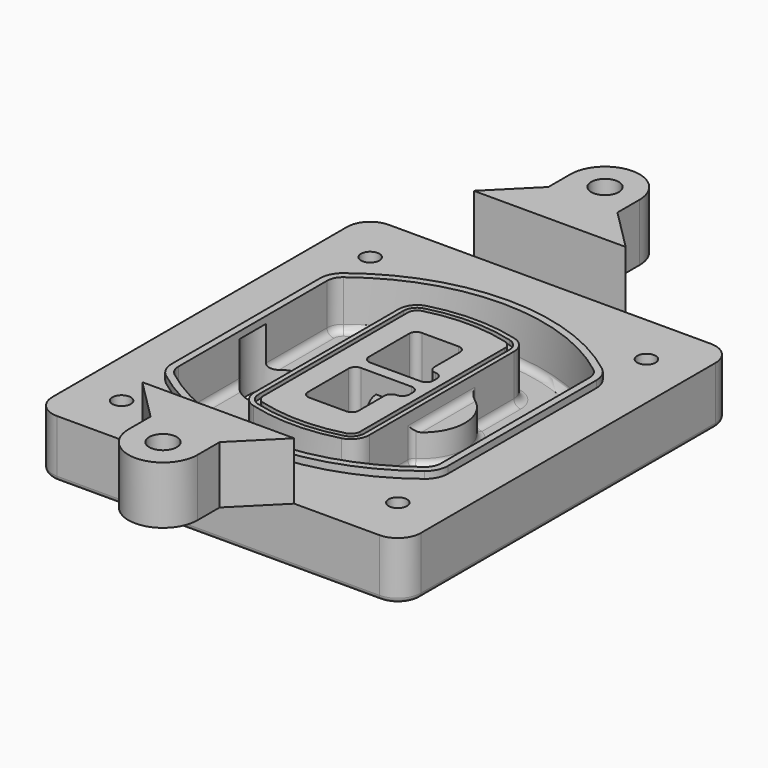
from build123d import *

# Parameters (mm, degrees)
F0_R      = 4
F1_DEPTH  = 25
F2_DEPTH  = 3
F3_DEPTH  = 18
F5_DEPTH  = 21
F6_DEPTH  = 2
F8_DEPTH  = 20
F9_DEPTH  = 16
F10_DEPTH = 25
F7_R      = 6
F7_R_2    = 4
F11_DEPTH = 6
F13_DEPTH = 9
F14_R     = 3
F15_R     = 2
F16_R     = 6
F17_DEPTH = 25


# Not quite as in the source:
# - a feature names something its author has since deleted; it is built from what else it names


with BuildPart() as f1:
    # F0 (on Top) → F1 (new body)
    with BuildSketch(Plane.XY):
        with BuildLine():
            ThreePointArc((-80, -80), (-77.0710678119, -87.0710678119), (-70, -90))
            Line((-70, -90), (70, -90))
            ThreePointArc((70, -90), (77.0710678119, -87.0710678119), (80, -80))
            Line((80, -80), (80, 80))
            ThreePointArc((80, 80), (77.0710678119, 87.0710678119), (70, 90))
            Line((70, 90), (-70, 90))
            ThreePointArc((-70, 90), (-77.0710678119, 87.0710678119), (-80, 80))
            Line((-80, 80), (-80, -80))
        make_face()
        with Locations((-60, -67.5)):
            Circle(F0_R, mode=Mode.SUBTRACT)
        with Locations((60, -67.5)):
            Circle(F0_R, mode=Mode.SUBTRACT)
        with Locations((-60, 67.5)):
            Circle(F0_R, mode=Mode.SUBTRACT)
        with BuildLine():
            ThreePointArc((-64, 40.2934422872), (-62.5820384798, 46.4328484224), (-58.6153846154, 51.3286200352))
            ThreePointArc((-58.6153846154, 51.3286200352), (0, 71.5), (58.6153846154, 51.3286200352))
            ThreePointArc((58.6153846154, 51.3286200352), (62.5820384798, 46.4328484224), (64, 40.2934422872))
            Line((64, 40.2934422872), (64, -40.2934422872))
            ThreePointArc((64, -40.2934422872), (62.5820384798, -46.4328484224), (58.6153846154, -51.3286200352))
            ThreePointArc((58.6153846154, -51.3286200352), (0, -71.5), (-58.6153846154, -51.3286200352))
            ThreePointArc((-58.6153846154, -51.3286200352), (-62.5820384798, -46.4328484224), (-64, -40.2934422872))
            Line((-64, -40.2934422872), (-64, 40.2934422872))
        make_face(mode=Mode.SUBTRACT)
        with Locations((60, 67.5)):
            Circle(F0_R, mode=Mode.SUBTRACT)
        with BuildLine():
            ThreePointArc((58.6153846154, 51.3286200352), (0, 71.5), (-58.6153846154, 51.3286200352))
            ThreePointArc((-58.6153846154, 51.3286200352), (-62.5820384798, 46.4328484224), (-64, 40.2934422872))
            Line((-64, 40.2934422872), (-64, -40.2934422872))
            ThreePointArc((-64, -40.2934422872), (-62.5820384798, -46.4328484224), (-58.6153846154, -51.3286200352))
            ThreePointArc((-58.6153846154, -51.3286200352), (0, -71.5), (58.6153846154, -51.3286200352))
            ThreePointArc((58.6153846154, -51.3286200352), (62.5820384798, -46.4328484224), (64, -40.2934422872))
            Line((64, -40.2934422872), (64, 40.2934422872))
            ThreePointArc((64, 40.2934422872), (62.5820384798, 46.4328484224), (58.6153846154, 51.3286200352))
        make_face()
        with BuildLine():
            Line((-60, -40.2934422872), (-60, 40.2934422872))
            ThreePointArc((-60, 40.2934422872), (-58.9871703427, 44.6787323838), (-56.1538461538, 48.1757121072))
            ThreePointArc((-56.1538461538, 48.1757121072), (0, 67.5), (56.1538461538, 48.1757121072))
            ThreePointArc((56.1538461538, 48.1757121072), (58.9871703427, 44.6787323838), (60, 40.2934422872))
            Line((60, 40.2934422872), (60, -40.2934422872))
            ThreePointArc((60, -40.2934422872), (58.9871703427, -44.6787323838), (56.1538461538, -48.1757121072))
            ThreePointArc((56.1538461538, -48.1757121072), (0, -67.5), (-56.1538461538, -48.1757121072))
            ThreePointArc((-56.1538461538, -48.1757121072), (-58.9871703427, -44.6787323838), (-60, -40.2934422872))
        make_face(mode=Mode.SUBTRACT)
        with BuildLine():
            ThreePointArc((-56.1538461538, 48.1757121072), (-58.9871703427, 44.6787323838), (-60, 40.2934422872))
            Line((-60, 40.2934422872), (-60, -40.2934422872))
            ThreePointArc((-60, -40.2934422872), (-58.9871703427, -44.6787323838), (-56.1538461538, -48.1757121072))
            ThreePointArc((-56.1538461538, -48.1757121072), (0, -67.5), (56.1538461538, -48.1757121072))
            ThreePointArc((56.1538461538, -48.1757121072), (58.9871703427, -44.6787323838), (60, -40.2934422872))
            Line((60, -40.2934422872), (60, 40.2934422872))
            ThreePointArc((60, 40.2934422872), (58.9871703427, 44.6787323838), (56.1538461538, 48.1757121072))
            ThreePointArc((56.1538461538, 48.1757121072), (0, 67.5), (-56.1538461538, 48.1757121072))
        make_face()
        with BuildLine():
            ThreePointArc((54.3076923077, 45.8110311612), (56.2910192399, 43.3631453548), (57, 40.2934422872))
            Line((57, 40.2934422872), (57, -40.2934422872))
            ThreePointArc((57, -40.2934422872), (56.2910192399, -43.3631453548), (54.3076923077, -45.8110311612))
            ThreePointArc((54.3076923077, -45.8110311612), (0, -64.5), (-54.3076923077, -45.8110311612))
            ThreePointArc((-54.3076923077, -45.8110311612), (-56.2910192399, -43.3631453548), (-57, -40.2934422872))
            Line((-57, -40.2934422872), (-57, 40.2934422872))
            ThreePointArc((-57, 40.2934422872), (-56.2910192399, 43.3631453548), (-54.3076923077, 45.8110311612))
            ThreePointArc((-54.3076923077, 45.8110311612), (0, 64.5), (54.3076923077, 45.8110311612))
        make_face(mode=Mode.SUBTRACT)
        with BuildLine():
            Line((57, -40.2934422872), (57, 40.2934422872))
            ThreePointArc((57, 40.2934422872), (56.2910192399, 43.3631453548), (54.3076923077, 45.8110311612))
            ThreePointArc((54.3076923077, 45.8110311612), (0, 64.5), (-54.3076923077, 45.8110311612))
            ThreePointArc((-54.3076923077, 45.8110311612), (-56.2910192399, 43.3631453548), (-57, 40.2934422872))
            Line((-57, 40.2934422872), (-57, -40.2934422872))
            ThreePointArc((-57, -40.2934422872), (-56.2910192399, -43.3631453548), (-54.3076923077, -45.8110311612))
            ThreePointArc((-54.3076923077, -45.8110311612), (0, -64.5), (54.3076923077, -45.8110311612))
            ThreePointArc((54.3076923077, -45.8110311612), (56.2910192399, -43.3631453548), (57, -40.2934422872))
        make_face()
    extrude(amount=-F1_DEPTH)

    # F0 (on Top) → F2 (join)
    with BuildSketch(Plane.XY):
        with BuildLine():
            ThreePointArc((-56.1538461538, 48.1757121072), (-58.9871703427, 44.6787323838), (-60, 40.2934422872))
            Line((-60, 40.2934422872), (-60, -40.2934422872))
            ThreePointArc((-60, -40.2934422872), (-58.9871703427, -44.6787323838), (-56.1538461538, -48.1757121072))
            ThreePointArc((-56.1538461538, -48.1757121072), (0, -67.5), (56.1538461538, -48.1757121072))
            ThreePointArc((56.1538461538, -48.1757121072), (58.9871703427, -44.6787323838), (60, -40.2934422872))
            Line((60, -40.2934422872), (60, 40.2934422872))
            ThreePointArc((60, 40.2934422872), (58.9871703427, 44.6787323838), (56.1538461538, 48.1757121072))
            ThreePointArc((56.1538461538, 48.1757121072), (0, 67.5), (-56.1538461538, 48.1757121072))
        make_face()
        with BuildLine():
            ThreePointArc((54.3076923077, 45.8110311612), (56.2910192399, 43.3631453548), (57, 40.2934422872))
            Line((57, 40.2934422872), (57, -40.2934422872))
            ThreePointArc((57, -40.2934422872), (56.2910192399, -43.3631453548), (54.3076923077, -45.8110311612))
            ThreePointArc((54.3076923077, -45.8110311612), (0, -64.5), (-54.3076923077, -45.8110311612))
            ThreePointArc((-54.3076923077, -45.8110311612), (-56.2910192399, -43.3631453548), (-57, -40.2934422872))
            Line((-57, -40.2934422872), (-57, 40.2934422872))
            ThreePointArc((-57, 40.2934422872), (-56.2910192399, 43.3631453548), (-54.3076923077, 45.8110311612))
            ThreePointArc((-54.3076923077, 45.8110311612), (0, 64.5), (54.3076923077, 45.8110311612))
        make_face(mode=Mode.SUBTRACT)
    extrude(amount=F2_DEPTH)

    # F0 (on Top) → F3 (cut)
    with BuildSketch(Plane.XY):
        with BuildLine():
            Line((57, -40.2934422872), (57, 40.2934422872))
            ThreePointArc((57, 40.2934422872), (56.2910192399, 43.3631453548), (54.3076923077, 45.8110311612))
            ThreePointArc((54.3076923077, 45.8110311612), (0, 64.5), (-54.3076923077, 45.8110311612))
            ThreePointArc((-54.3076923077, 45.8110311612), (-56.2910192399, 43.3631453548), (-57, 40.2934422872))
            Line((-57, 40.2934422872), (-57, -40.2934422872))
            ThreePointArc((-57, -40.2934422872), (-56.2910192399, -43.3631453548), (-54.3076923077, -45.8110311612))
            ThreePointArc((-54.3076923077, -45.8110311612), (0, -64.5), (54.3076923077, -45.8110311612))
            ThreePointArc((54.3076923077, -45.8110311612), (56.2910192399, -43.3631453548), (57, -40.2934422872))
        make_face()
    extrude(amount=-F3_DEPTH, mode=Mode.SUBTRACT)

    # F4 (on face) → F5 (join, through all)
    with BuildSketch(Plane.XY.offset(3)):
        with BuildLine():
            ThreePointArc((-25, -39.2465276821), (-23.3511545998, -44.1109737193), (-19.0842911877, -46.9702398883))
            ThreePointArc((-19.0842911877, -46.9702398883), (0, -49.5), (19.0842911877, -46.9702398883))
            ThreePointArc((19.0842911877, -46.9702398883), (23.3511545998, -44.1109737193), (25, -39.2465276821))
            Line((25, -39.2465276821), (25, 39.2465276821))
            ThreePointArc((25, 39.2465276821), (23.3511545998, 44.1109737193), (19.0842911877, 46.9702398883))
            ThreePointArc((19.0842911877, 46.9702398883), (0, 49.5), (-19.0842911877, 46.9702398883))
            ThreePointArc((-19.0842911877, 46.9702398883), (-23.3511545998, 44.1109737193), (-25, 39.2465276821))
            Line((-25, 39.2465276821), (-25, -39.2465276821))
        make_face()
        with BuildLine():
            ThreePointArc((18.5632183908, 45.0393118368), (21.7633659499, 42.89486221), (23, 39.2465276821))
            Line((23, 39.2465276821), (23, -39.2465276821))
            ThreePointArc((23, -39.2465276821), (21.7633659499, -42.89486221), (18.5632183908, -45.0393118368))
            ThreePointArc((18.5632183908, -45.0393118368), (0, -47.5), (-18.5632183908, -45.0393118368))
            ThreePointArc((-18.5632183908, -45.0393118368), (-21.7633659499, -42.89486221), (-23, -39.2465276821))
            Line((-23, -39.2465276821), (-23, 39.2465276821))
            ThreePointArc((-23, 39.2465276821), (-21.7633659499, 42.89486221), (-18.5632183908, 45.0393118368))
            ThreePointArc((-18.5632183908, 45.0393118368), (0, 47.5), (18.5632183908, 45.0393118368))
        make_face(mode=Mode.SUBTRACT)
        with BuildLine():
            Line((23, -39.2465276821), (23, 39.2465276821))
            ThreePointArc((23, 39.2465276821), (21.7633659499, 42.89486221), (18.5632183908, 45.0393118368))
            ThreePointArc((18.5632183908, 45.0393118368), (0, 47.5), (-18.5632183908, 45.0393118368))
            ThreePointArc((-18.5632183908, 45.0393118368), (-21.7633659499, 42.89486221), (-23, 39.2465276821))
            Line((-23, 39.2465276821), (-23, -39.2465276821))
            ThreePointArc((-23, -39.2465276821), (-21.7633659499, -42.89486221), (-18.5632183908, -45.0393118368))
            ThreePointArc((-18.5632183908, -45.0393118368), (0, -47.5), (18.5632183908, -45.0393118368))
            ThreePointArc((18.5632183908, -45.0393118368), (21.7633659499, -42.89486221), (23, -39.2465276821))
        make_face()
        with BuildLine():
            ThreePointArc((18.0421455939, 43.1083837852), (20.1755772999, 41.6787507007), (21, 39.2465276821))
            Line((21, 39.2465276821), (21, -39.2465276821))
            ThreePointArc((21, -39.2465276821), (20.1755772999, -41.6787507007), (18.0421455939, -43.1083837852))
            ThreePointArc((18.0421455939, -43.1083837852), (0, -45.5), (-18.0421455939, -43.1083837852))
            ThreePointArc((-18.0421455939, -43.1083837852), (-20.1755772999, -41.6787507007), (-21, -39.2465276821))
            Line((-21, -39.2465276821), (-21, 39.2465276821))
            ThreePointArc((-21, 39.2465276821), (-20.1755772999, 41.6787507007), (-18.0421455939, 43.1083837852))
            ThreePointArc((-18.0421455939, 43.1083837852), (0, 45.5), (18.0421455939, 43.1083837852))
        make_face(mode=Mode.SUBTRACT)
        with BuildLine():
            Line((21, -39.2465276821), (21, 39.2465276821))
            ThreePointArc((21, 39.2465276821), (20.1755772999, 41.6787507007), (18.0421455939, 43.1083837852))
            ThreePointArc((18.0421455939, 43.1083837852), (0, 45.5), (-18.0421455939, 43.1083837852))
            ThreePointArc((-18.0421455939, 43.1083837852), (-20.1755772999, 41.6787507007), (-21, 39.2465276821))
            Line((-21, 39.2465276821), (-21, -39.2465276821))
            ThreePointArc((-21, -39.2465276821), (-20.1755772999, -41.6787507007), (-18.0421455939, -43.1083837852))
            ThreePointArc((-18.0421455939, -43.1083837852), (0, -45.5), (18.0421455939, -43.1083837852))
            ThreePointArc((18.0421455939, -43.1083837852), (20.1755772999, -41.6787507007), (21, -39.2465276821))
        make_face()
        with BuildLine():
            Line((-8, -2.5), (14, -2.5))
            ThreePointArc((14, -2.5), (16.1213203436, -3.3786796564), (17, -5.5))
            Line((17, -5.5), (17, -7.5))
            ThreePointArc((17, -7.5), (16.1213203436, -9.6213203436), (14, -10.5))
            ThreePointArc((14, -10.5), (11.8786796564, -11.3786796564), (11, -13.5))
            Line((11, -13.5), (11, -27.5))
            ThreePointArc((11, -27.5), (10.1213203436, -29.6213203436), (8, -30.5))
            Line((8, -30.5), (-8, -30.5))
            ThreePointArc((-8, -30.5), (-10.1213203436, -29.6213203436), (-11, -27.5))
            Line((-11, -27.5), (-11, -5.5))
            ThreePointArc((-11, -5.5), (-10.1213203436, -3.3786796564), (-8, -2.5))
        make_face(mode=Mode.SUBTRACT)
        with BuildLine():
            ThreePointArc((-8, 2.5), (-10.1213203436, 3.3786796564), (-11, 5.5))
            Line((-11, 5.5), (-11, 27.5))
            ThreePointArc((-11, 27.5), (-10.1213203436, 29.6213203436), (-8, 30.5))
            Line((-8, 30.5), (8, 30.5))
            ThreePointArc((8, 30.5), (10.1213203436, 29.6213203436), (11, 27.5))
            Line((11, 27.5), (11, 13.5))
            ThreePointArc((11, 13.5), (11.8786796564, 11.3786796564), (14, 10.5))
            ThreePointArc((14, 10.5), (16.1213203436, 9.6213203436), (17, 7.5))
            Line((17, 7.5), (17, 5.5))
            ThreePointArc((17, 5.5), (16.1213203436, 3.3786796564), (14, 2.5))
            Line((14, 2.5), (-8, 2.5))
        make_face(mode=Mode.SUBTRACT)
    extrude(amount=-F5_DEPTH)

    # F4 (on face) → F6 (cut)
    with BuildSketch(Plane.XY.offset(3)):
        with BuildLine():
            Line((23, -39.2465276821), (23, 39.2465276821))
            ThreePointArc((23, 39.2465276821), (21.7633659499, 42.89486221), (18.5632183908, 45.0393118368))
            ThreePointArc((18.5632183908, 45.0393118368), (0, 47.5), (-18.5632183908, 45.0393118368))
            ThreePointArc((-18.5632183908, 45.0393118368), (-21.7633659499, 42.89486221), (-23, 39.2465276821))
            Line((-23, 39.2465276821), (-23, -39.2465276821))
            ThreePointArc((-23, -39.2465276821), (-21.7633659499, -42.89486221), (-18.5632183908, -45.0393118368))
            ThreePointArc((-18.5632183908, -45.0393118368), (0, -47.5), (18.5632183908, -45.0393118368))
            ThreePointArc((18.5632183908, -45.0393118368), (21.7633659499, -42.89486221), (23, -39.2465276821))
        make_face()
        with BuildLine():
            ThreePointArc((18.0421455939, 43.1083837852), (20.1755772999, 41.6787507007), (21, 39.2465276821))
            Line((21, 39.2465276821), (21, -39.2465276821))
            ThreePointArc((21, -39.2465276821), (20.1755772999, -41.6787507007), (18.0421455939, -43.1083837852))
            ThreePointArc((18.0421455939, -43.1083837852), (0, -45.5), (-18.0421455939, -43.1083837852))
            ThreePointArc((-18.0421455939, -43.1083837852), (-20.1755772999, -41.6787507007), (-21, -39.2465276821))
            Line((-21, -39.2465276821), (-21, 39.2465276821))
            ThreePointArc((-21, 39.2465276821), (-20.1755772999, 41.6787507007), (-18.0421455939, 43.1083837852))
            ThreePointArc((-18.0421455939, 43.1083837852), (0, 45.5), (18.0421455939, 43.1083837852))
        make_face(mode=Mode.SUBTRACT)
    extrude(amount=-F6_DEPTH, mode=Mode.SUBTRACT)

    # F7 (on face) → F8 (join)
    with BuildSketch(Plane(origin=(0, 0, -25), x_dir=(1, 0, 0), z_dir=(0, 0, -1))):
        with BuildLine():
            ThreePointArc((3.28842436, 0), (16.7567035675, 13.4682792075), (30.224982775, 0))
            Line((30.224982775, 0), (35.224982775, 0))
            ThreePointArc((35.224982775, 0), (16.7567035675, 18.4682792075), (-1.71157564, 0))
            Line((-1.71157564, 0), (3.28842436, 0))
        make_face()
        with BuildLine():
            Line((3.28842436, 0), (30.224982775, 0))
            ThreePointArc((30.224982775, 0), (16.7567035675, 13.4682792075), (3.28842436, 0))
        make_face()
        with BuildLine():
            ThreePointArc((3.28842436, 0), (16.7567035675, -13.4682792075), (30.224982775, 0))
            Line((30.224982775, 0), (3.28842436, 0))
        make_face()
        with BuildLine():
            Line((35.224982775, 0), (30.224982775, 0))
            ThreePointArc((30.224982775, 0), (16.7567035675, -13.4682792075), (3.28842436, 0))
            Line((3.28842436, 0), (-1.71157564, 0))
            ThreePointArc((-1.71157564, 0), (16.7567035675, -18.4682792075), (35.224982775, 0))
        make_face()
    extrude(amount=-F8_DEPTH)

    # F7 (on face) → F9 (cut)
    with BuildSketch(Plane(origin=(0, 0, -25), x_dir=(1, 0, 0), z_dir=(0, 0, -1))):
        with BuildLine():
            Line((3.28842436, 0), (30.224982775, 0))
            ThreePointArc((30.224982775, 0), (16.7567035675, 13.4682792075), (3.28842436, 0))
        make_face()
        with BuildLine():
            ThreePointArc((3.28842436, 0), (16.7567035675, -13.4682792075), (30.224982775, 0))
            Line((30.224982775, 0), (3.28842436, 0))
        make_face()
    extrude(amount=-F9_DEPTH, mode=Mode.SUBTRACT)

    # F7 (on face) → F10 (cut)
    with BuildSketch(Plane(origin=(0, 0, -25), x_dir=(1, 0, 0), z_dir=(0, 0, -1))):
        with BuildLine():
            Line((-59.0318229325, 0), (-32.0952645175, 0))
            ThreePointArc((-32.0952645175, 0), (-45.563543725, 13.4682792075), (-59.0318229325, 0))
        make_face()
        with BuildLine():
            ThreePointArc((-59.0318229325, 0), (-45.563543725, -13.4682792075), (-32.0952645175, 0))
            Line((-32.0952645175, 0), (-59.0318229325, 0))
        make_face()
    extrude(amount=-F10_DEPTH, mode=Mode.SUBTRACT)

    # F7 (on face) → F11 (cut)
    with BuildSketch(Plane(origin=(0, 0, -25), x_dir=(1, 0, 0), z_dir=(0, 0, -1))):
        with Locations((60, -67.5)):
            Circle(F7_R)
        with Locations((60, -67.5)):
            Circle(F7_R_2, mode=Mode.SUBTRACT)
        with Locations((-60, -67.5)):
            Circle(F7_R)
        with Locations((-60, -67.5)):
            Circle(F7_R_2, mode=Mode.SUBTRACT)
        with Locations((-60, 67.5)):
            Circle(F7_R)
        with Locations((-60, 67.5)):
            Circle(F7_R_2, mode=Mode.SUBTRACT)
        with Locations((60, 67.5)):
            Circle(F7_R)
        with Locations((60, 67.5)):
            Circle(F7_R_2, mode=Mode.SUBTRACT)
    extrude(amount=-F11_DEPTH, mode=Mode.SUBTRACT)

    # F12 (on face) → F13 (cut, through all)
    with BuildSketch(Plane(origin=(0, 0, -9), x_dir=(1, 0, 0), z_dir=(0, 0, -1))):
        with BuildLine():
            Line((11, 13.5), (11, 17.5481537753))
            ThreePointArc((11, 17.5481537753), (2.5696536419, 11.8239143813), (-1.5415842455, 2.5))
            Line((-1.5415842455, 2.5), (3.5224848595, 2.5))
            ThreePointArc((3.5224848595, 2.5), (6.1857188154, 8.3455872281), (11.2536447004, 12.2927168648))
            ThreePointArc((11.2536447004, 12.2927168648), (11.0640958889, 12.8831798879), (11, 13.5))
        make_face()
        with BuildLine():
            ThreePointArc((11.2536447004, -12.2927168648), (6.1857188154, -8.3455872281), (3.5224848595, -2.5))
            Line((3.5224848595, -2.5), (-1.5415842455, -2.5))
            ThreePointArc((-1.5415842455, -2.5), (2.5696536419, -11.8239143813), (11, -17.5481537753))
            Line((11, -17.5481537753), (11, -13.5))
            ThreePointArc((11, -13.5), (11.0640958889, -12.8831798879), (11.2536447004, -12.2927168648))
        make_face()
        with BuildLine():
            ThreePointArc((11.2536447004, 12.2927168648), (6.1857188154, 8.3455872281), (3.5224848595, 2.5))
            Line((3.5224848595, 2.5), (14, 2.5))
            ThreePointArc((14, 2.5), (16.1213203436, 3.3786796564), (17, 5.5))
            Line((17, 5.5), (17, 7.5))
            ThreePointArc((17, 7.5), (16.1213203436, 9.6213203436), (14, 10.5))
            ThreePointArc((14, 10.5), (12.3601599782, 10.9878446101), (11.2536447004, 12.2927168648))
        make_face()
        with BuildLine():
            Line((14, -2.5), (3.5224848595, -2.5))
            ThreePointArc((3.5224848595, -2.5), (6.1857188154, -8.3455872281), (11.2536447004, -12.2927168648))
            ThreePointArc((11.2536447004, -12.2927168648), (12.3601599782, -10.9878446101), (14, -10.5))
            ThreePointArc((14, -10.5), (16.1213203436, -9.6213203436), (17, -7.5))
            Line((17, -7.5), (17, -5.5))
            ThreePointArc((17, -5.5), (16.1213203436, -3.3786796564), (14, -2.5))
        make_face()
    extrude(amount=F13_DEPTH, mode=Mode.SUBTRACT)

    # F14
    f14_edges = [f1.edges().sort_by_distance(p)[0] for p in [
        (-57, -23.703476, -18),
        (-57, 23.703476, -18),
        (25, 0, -5),
        (25, 16.526506, -11.5),
        (25, -16.526506, -11.5),
        (25, -27.886517, -18),
        (35.224983, 0, -18),
    ]]
    fillet(f14_edges, radius=F14_R)

    # F15
    f15_edges = [f1.edges().sort_by_distance(p)[0] for p in [
        (0, -90, -25),
    ]]
    fillet(f15_edges, radius=F15_R)


with BuildPart() as f17:
    # F16 (on face) → F17 (new body)
    with BuildSketch(Plane.XY):
        with BuildLine():
            Line((-15, 108), (-33, 90))
            Line((-33, 90), (33, 90))
            Line((33, 90), (15, 108))
            Line((15, 108), (15, 120))
            ThreePointArc((15, 120), (0, 135), (-15, 120))
            Line((-15, 120), (-15, 108))
        make_face()
        with Locations((0, 120)):
            Circle(F16_R, mode=Mode.SUBTRACT)
    extrude(amount=F17_DEPTH)


with BuildPart() as f17b:
    # F16 (on face) → F17, piece 2 (new body)
    with BuildSketch(Plane.XY):
        with BuildLine():
            Line((33, -90), (-33, -90))
            Line((-33, -90), (-15, -108))
            Line((-15, -108), (-15, -120))
            ThreePointArc((-15, -120), (0, -135), (15, -120))
            Line((15, -120), (15, -108))
            Line((15, -108), (33, -90))
        make_face()
        with Locations((0, -120)):
            Circle(F16_R, mode=Mode.SUBTRACT)
    extrude(amount=F17_DEPTH)


solid = Compound([f1.part, f17.part, f17b.part])
